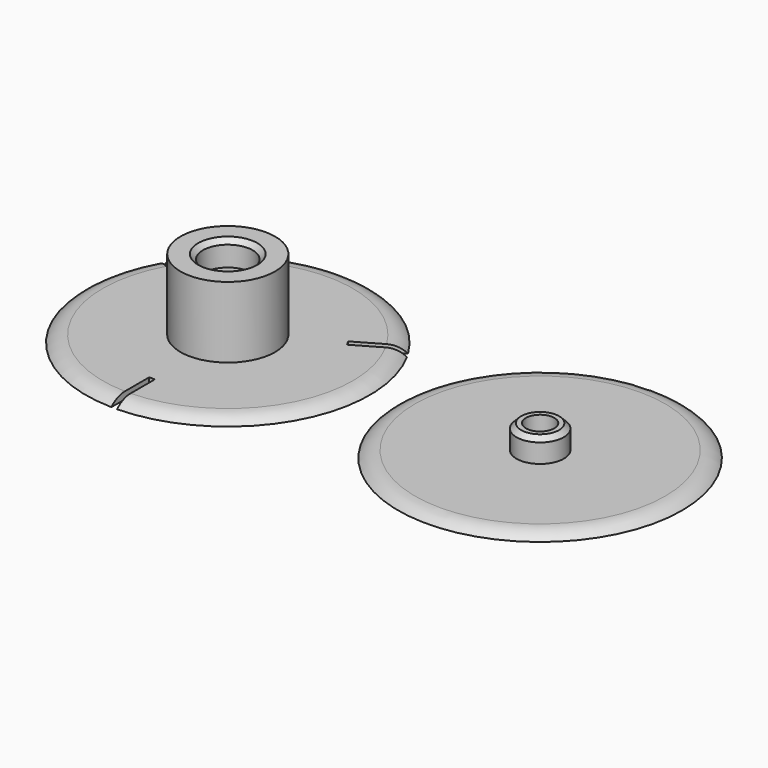
from build123d import *

# Parameters (mm, degrees)
F0_R       = 30
F1_DEPTH   = 1.5
F3_R       = 10
F4_DEPTH   = 15
F5_R       = 5
F6_DEPTH   = 5
F7_R       = 5.25
F8_DEPTH   = 5.25
F9_R       = 3
F11_DEPTH  = 25
F10_R      = 3
F12_DEPTH  = 25
F13_R      = 0.75
F14_DEPTH  = 30.001
F15_W      = 1.2
F15_H      = 20
F16_DEPTH  = 25
F17_SIZE   = 1
F17_2_SIZE = 1


# Not quite as in the source:
# - a fillet or chamfer that OpenCascade refuses, or shapes differently, is made with other operations: its cross-section is extruded or revolved along the edge and cut away or added


with BuildPart() as f1:
    # F0 (on Top) → F1 (new body)
    with BuildSketch(Plane.XY):
        with Locations((-33, 0)):
            Circle(F0_R)
    extrude(amount=F1_DEPTH)

    # F2: fillet of radius 5 on 1 edges, made by hand

    # F2_s1 → F2_t2 (revolve, cut)
    with BuildSketch(Plane.XZ):
        with BuildLine():
            ThreePointArc((-3, 0), (-4.6342225412, 1.1097722286), (-6.5707142143, 1.5))
            Line((-6.5707142143, 1.5), (-3, 1.5))
            Line((-3, 1.5), (-3, 0))
        make_face()
    revolve(axis=Axis((-33, 0, 1.5), (0, 0, 1)), mode=Mode.SUBTRACT)

    # F3 (on face) → F4 (join)
    with BuildSketch(Plane.XY.offset(1.5)):
        with Locations((-33, 0)):
            Circle(F3_R)
    extrude(amount=F4_DEPTH)

    # F7 (on face) → F8 (cut)
    with BuildSketch(Plane.XY.offset(16.5)):
        with Locations((-33, 0)):
            Circle(F7_R)
    extrude(amount=-F8_DEPTH, mode=Mode.SUBTRACT)

    # F10 (on face) → F12 (cut)
    with BuildSketch(Plane(origin=(0, 0, 0), x_dir=(1, 0, 0), z_dir=(0, 0, -1))):
        with Locations((-33, 0)):
            Circle(F10_R)
    extrude(amount=-F12_DEPTH, mode=Mode.SUBTRACT)

    # F13 (on Front) → F14 (cut, through all)
    with BuildSketch(Plane.XZ):
        with Locations((-33, 4)):
            Circle(F13_R)
    extrude(amount=-F14_DEPTH, mode=Mode.SUBTRACT)

    # F15 (on face) → F16 (cut)
    with BuildSketch(Plane(origin=(0, 0, 0), x_dir=(1, 0, 0), z_dir=(0, 0, -1))):
        with Locations((-33, 30)):
            Rectangle(F15_W, F15_H)
        Polygon((-67.3410161514, -20.5196152423), (-50.0205080757, -10.5196152423), (-50.6205080757, -9.4803847577), (-67.9410161514, -19.4803847577), align=None)
        Polygon((1.9410161514, -19.4803847577), (-15.3794919243, -9.4803847577), (-15.9794919243, -10.5196152423), (1.3410161514, -20.5196152423), align=None)
    extrude(amount=-F16_DEPTH, mode=Mode.SUBTRACT)

    # F17
    f17_edges = [f1.edges().sort_by_distance(p)[0] for p in [
        (-38.25, 0, 16.5),
    ]]
    chamfer(f17_edges, length=F17_SIZE)


with BuildPart() as f1b:
    # F0 (on Top) → F1, piece 2 (new body)
    with BuildSketch(Plane.XY):
        with Locations((33, 0)):
            Circle(F0_R)
    extrude(amount=F1_DEPTH)

    # F2#2: fillet of radius 5 on 1 edges, made by hand

    # F2_2_s1 → F2_2_t2 (revolve, cut)
    with BuildSketch(Plane.XZ):
        with BuildLine():
            ThreePointArc((63, 0), (61.3657774588, 1.1097722286), (59.4292857857, 1.5))
            Line((59.4292857857, 1.5), (63, 1.5))
            Line((63, 1.5), (63, 0))
        make_face()
    revolve(axis=Axis((33, 0, 1.5), (0, 0, 1)), mode=Mode.SUBTRACT)

    # F5 (on face) → F6 (join)
    with BuildSketch(Plane.XY.offset(1.5)):
        with Locations((33, 0)):
            Circle(F5_R)
    extrude(amount=F6_DEPTH)

    # F9 (on face) → F11 (cut)
    with BuildSketch(Plane(origin=(0, 0, 0), x_dir=(1, 0, 0), z_dir=(0, 0, -1))):
        with Locations((33, 0)):
            Circle(F9_R)
    extrude(amount=-F11_DEPTH, mode=Mode.SUBTRACT)

    # F17#2
    f17_2_edges = [f1b.edges().sort_by_distance(p)[0] for p in [
        (28, 0, 6.5),
    ]]
    chamfer(f17_2_edges, length=F17_2_SIZE)


solid = Compound([f1.part, f1b.part])
